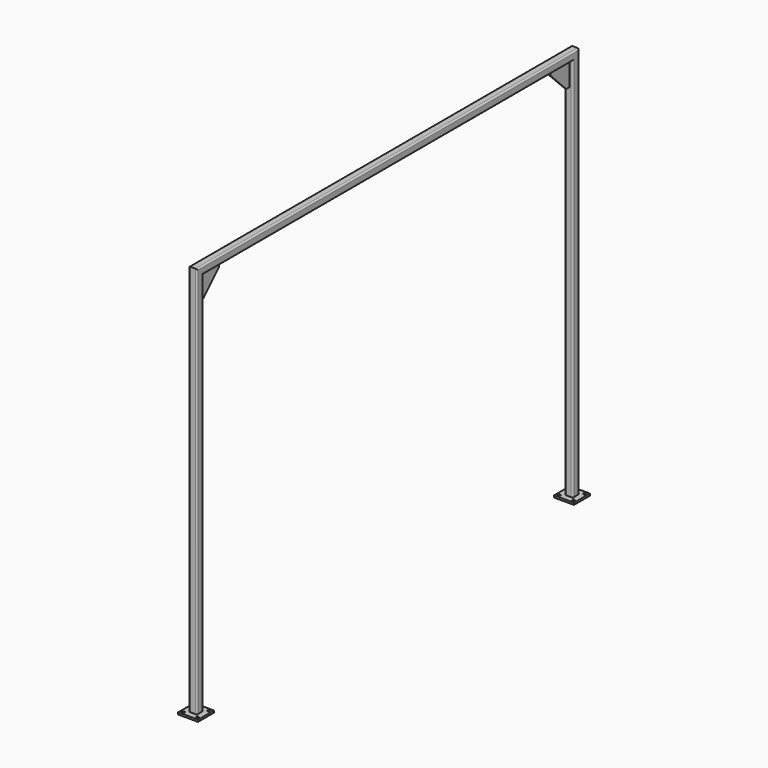
from build123d import *

# Parameters (mm, degrees)
F3_W      = 127
F3_H      = 127
F4_DEPTH  = 12.7
F6_D      = 14.2875
F10_DEPTH = 4.7625


# Not quite as in the source:
# - a length typed as a fraction of an inch, garbled in the dataset ("3 / 203.2 mm" for 3/8 in), is restored
# - a feature names something its author has since deleted; it is built from what else it names


with BuildPart() as f2:
    # F2: sweep along a path in F0
    with BuildLine(Plane.YZ) as f2_path:
        Line((-1524, 0), (-1524, 2501.9))
        Line((-1524, 2501.9), (1524, 2501.9))
        Line((1524, 2501.9), (1524, 0))
    # F1 (on Top) → F2 (sweep)
    with BuildSketch(Plane.XY):
        with BuildLine():
            Line((-15.748, -1524), (0, -1524))
            Line((0, -1524), (15.748, -1524))
            ThreePointArc((15.748, -1524), (22.572994652, -1521.172994652), (25.4, -1514.348))
            Line((25.4, -1514.348), (25.4, -1482.852))
            ThreePointArc((25.4, -1482.852), (22.572994652, -1476.027005348), (15.748, -1473.2))
            Line((15.748, -1473.2), (-15.748, -1473.2))
            ThreePointArc((-15.748, -1473.2), (-22.572994652, -1476.027005348), (-25.4, -1482.852))
            Line((-25.4, -1482.852), (-25.4, -1514.348))
            ThreePointArc((-25.4, -1514.348), (-22.572994652, -1521.172994652), (-15.748, -1524))
        make_face()
        with BuildLine():
            Line((0, -1519.2375), (-15.748, -1519.2375))
            ThreePointArc((-15.748, -1519.2375), (-19.2053986066, -1517.8053986066), (-20.6375, -1514.348))
            Line((-20.6375, -1514.348), (-20.6375, -1482.852))
            ThreePointArc((-20.6375, -1482.852), (-19.2053986066, -1479.3946013934), (-15.748, -1477.9625))
            Line((-15.748, -1477.9625), (15.748, -1477.9625))
            ThreePointArc((15.748, -1477.9625), (19.2053986066, -1479.3946013934), (20.6375, -1482.852))
            Line((20.6375, -1482.852), (20.6375, -1514.348))
            ThreePointArc((20.6375, -1514.348), (19.2053986066, -1517.8053986066), (15.748, -1519.2375))
            Line((15.748, -1519.2375), (0, -1519.2375))
        make_face(mode=Mode.SUBTRACT)
    sweep(path=f2_path.line, transition=Transition.RIGHT)

    # F3 (on face) → F4 (join)
    with BuildSketch(Plane(origin=(0, 0, 0), x_dir=(1, 0, 0), z_dir=(0, 0, -1))):
        with Locations((0, 1498.6)):
            Rectangle(F3_W, F3_H)
    extrude(amount=F4_DEPTH)

    # F6 (through all)
    with Locations(Plane(origin=(0, 0, -12.7), x_dir=(1, 0, 0), z_dir=(0, 0, -1))):
        with Locations((-44.45, 1454.15), (-44.45, 1543.05), (44.45, 1543.05), (44.45, 1454.15)):
            Hole(F6_D / 2)


with BuildPart() as f7_1:
    # F7: instance of F2
    add(f2.part.mirror(Plane.XZ))


with BuildPart() as f2_1:
    add(f2.part)

    add(f7_1.part)  # F10 merges F7_1
    # F9 (on mid) → F10 (join, symmetric)
    with BuildSketch(Plane.YZ):
        Polygon((-1320.8, 2451.1), (-1473.2, 2451.1), (-1473.2, 2298.7), (-1447.8, 2298.7), (-1320.8, 2425.7), align=None)
    extrude(amount=F10_DEPTH, both=True)

    # F11: F2 across plane


with BuildPart() as f2_2:
    add(f2_1.part)
    add(f2_1.part.mirror(Plane.XZ))


solid = f2_2.part
